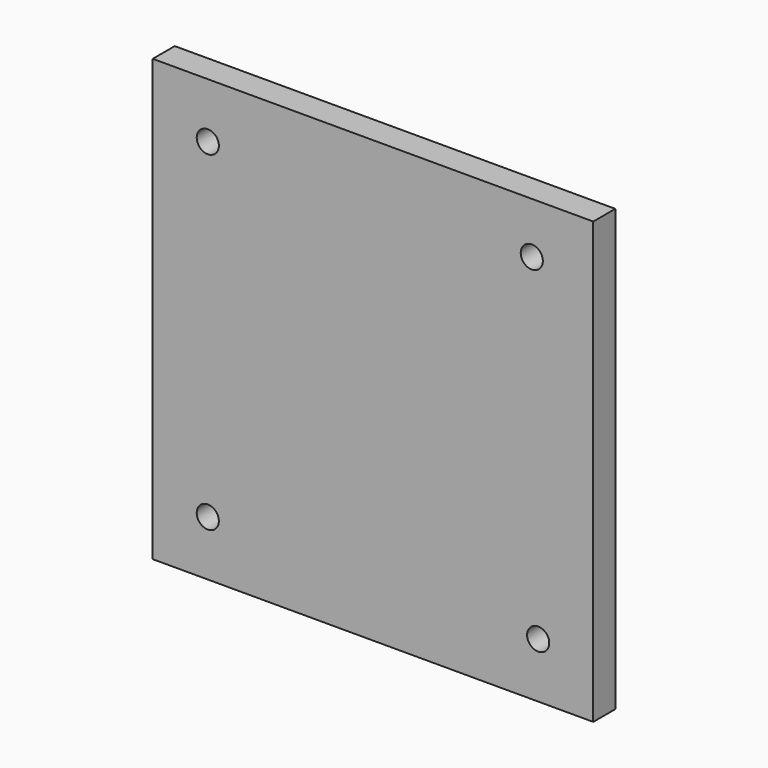
from build123d import *

# Parameters (mm, degrees)
F0_W     = 101.6
F0_H     = 101.6
F1_DEPTH = 6.35
F2_D     = 5.1054
F3_D     = 5.1054


# Not quite as in the source:
# - a feature names something its author has since deleted; it is built from what else it names


with BuildPart() as f1:
    # F0 (on Front) → F1 (new body)
    with BuildSketch(Plane.XZ):
        Rectangle(F0_W, F0_H)
    extrude(amount=F1_DEPTH)

    # F2 (through all)
    with Locations(Plane(origin=(0, 0, 0), x_dir=(1, 0, 0), z_dir=(0, 1, 0))):
        with Locations((-38.1, -38.1), (38.1, 38.1), (-38.1, 38.1)):
            Hole(F2_D / 2)

    # F3 (through all)
    with Locations(Plane(origin=(0, 0, 0), x_dir=(1, 0, 0), z_dir=(0, 1, 0))):
        with Locations((36.6242937744, -38.9907881618)):
            Hole(F3_D / 2)


solid = f1.part
